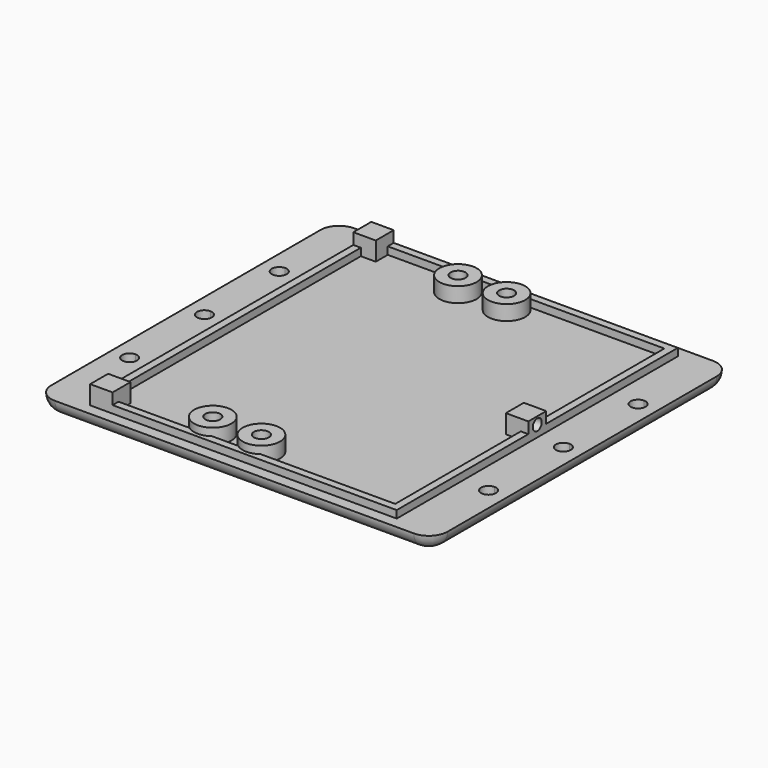
from build123d import *

# Parameters (mm, degrees)
F0_W          = 106
F0_H          = 100
F1_DEPTH      = 4
F2_W          = 82
F2_H          = 94
F2_W_2        = 78
F2_H_2        = 90
F5_DEPTH      = 2
F6_DEPTH      = 25
F4_R          = 5
F4_R_2        = 2
F7_DEPTH      = 4
F8_W          = 6
F8_H          = 6
F9_DEPTH      = 5
F10_R         = 1.5
F11_DEPTH     = 5
F12_W         = 6
F12_H         = 6
F13_DEPTH     = 5
F14_R         = 1.5
F15_DEPTH     = 5
F16_R         = 5
F17_T1_DEPTH  = 90
F17_T3_DEPTH  = 96
F17_T6_ANGLE  = 90
F17_T8_ANGLE  = 90
F17_T10_ANGLE = 90
F17_T12_ANGLE = 90


# Not quite as in the source:
# - a fillet or chamfer that OpenCascade refuses, or shapes differently, is made with other operations: its cross-section is extruded or revolved along the edge and cut away or added


with BuildPart() as f1:
    # F0 (on Top) → F1 (new body)
    with BuildSketch(Plane.XY):
        with Locations((-29.9393483698, 26.8405017372)):
            Rectangle(F0_W, F0_H)
    extrude(amount=F1_DEPTH)

    # F2 (on face) → F5 (join)
    with BuildSketch(Plane.XY.offset(4)):
        with Locations((-29.9393483698, 26.8405017372)):
            Rectangle(F2_W, F2_H)
        with Locations((-29.9393483698, 26.8405017372)):
            Rectangle(F2_W_2, F2_H_2, mode=Mode.SUBTRACT)
    extrude(amount=F5_DEPTH)

    # F3 (on face) → F6 (cut)
    with BuildSketch(Plane.XY.offset(4)):
        with BuildLine():
            ThreePointArc((-77.9393483698, 49.7999965698), (-76.5251348075, 50.3857830074), (-75.9393483698, 51.7999965698))
            ThreePointArc((-75.9393483698, 51.7999965698), (-76.5251348075, 53.2142101321), (-77.9393483698, 53.7999965698))
            Line((-77.9393483698, 53.7999965698), (-77.9393483698, 51.7999965698))
            Line((-77.9393483698, 51.7999965698), (-77.9393483698, 49.7999965698))
        make_face()
        with BuildLine():
            ThreePointArc((-75.9393483698, 1.7999965698), (-76.5251348075, 3.2142101321), (-77.9393483698, 3.7999965698))
            Line((-77.9393483698, 3.7999965698), (-77.9393483698, 1.7999965698))
            Line((-77.9393483698, 1.7999965698), (-77.9393483698, -0.2000034302))
            ThreePointArc((-77.9393483698, -0.2000034302), (-76.5251348075, 0.3857830074), (-75.9393483698, 1.7999965698))
        make_face()
        with BuildLine():
            Line((-77.9393483698, 1.7999965698), (-77.9393483698, 3.7999965698))
            ThreePointArc((-77.9393483698, 3.7999965698), (-79.9393483698, 1.7999965698), (-77.9393483698, -0.2000034302))
            Line((-77.9393483698, -0.2000034302), (-77.9393483698, 1.7999965698))
        make_face()
        with BuildLine():
            ThreePointArc((-75.9393483698, 26.7999965698), (-76.5251348075, 28.2142101321), (-77.9393483698, 28.7999965698))
            Line((-77.9393483698, 28.7999965698), (-77.9393483698, 26.7999965698))
            Line((-77.9393483698, 26.7999965698), (-77.9393483698, 24.7999965698))
            ThreePointArc((-77.9393483698, 24.7999965698), (-76.5251348075, 25.3857830074), (-75.9393483698, 26.7999965698))
        make_face()
        with BuildLine():
            Line((-77.9393483698, 26.7999965698), (-77.9393483698, 28.7999965698))
            ThreePointArc((-77.9393483698, 28.7999965698), (-79.9393483698, 26.7999965698), (-77.9393483698, 24.7999965698))
            Line((-77.9393483698, 24.7999965698), (-77.9393483698, 26.7999965698))
        make_face()
        with BuildLine():
            Line((-77.9393483698, 51.7999965698), (-77.9393483698, 53.7999965698))
            ThreePointArc((-77.9393483698, 53.7999965698), (-79.9393483698, 51.7999965698), (-77.9393483698, 49.7999965698))
            Line((-77.9393483698, 49.7999965698), (-77.9393483698, 51.7999965698))
        make_face()
        with BuildLine():
            ThreePointArc((18.0606516302, 49.7999965698), (19.4748651925, 50.3857830074), (20.0606516302, 51.7999965698))
            ThreePointArc((20.0606516302, 51.7999965698), (19.4748651925, 53.2142101321), (18.0606516302, 53.7999965698))
            Line((18.0606516302, 53.7999965698), (18.0606516302, 51.7999965698))
            Line((18.0606516302, 51.7999965698), (18.0606516302, 49.7999965698))
        make_face()
        with BuildLine():
            ThreePointArc((20.0606516302, 1.7999965698), (19.4748651925, 3.2142101321), (18.0606516302, 3.7999965698))
            ThreePointArc((18.0606516302, 3.7999965698), (16.6464380678, 0.3857830074), (20.0606516302, 1.7999965698))
        make_face()
        with BuildLine():
            ThreePointArc((20.0606516302, 26.7999965698), (19.4748651925, 28.2142101321), (18.0606516302, 28.7999965698))
            Line((18.0606516302, 28.7999965698), (18.0606516302, 26.7999965698))
            Line((18.0606516302, 26.7999965698), (18.0606516302, 24.7999965698))
            ThreePointArc((18.0606516302, 24.7999965698), (19.4748651925, 25.3857830074), (20.0606516302, 26.7999965698))
        make_face()
        with BuildLine():
            Line((18.0606516302, 26.7999965698), (18.0606516302, 28.7999965698))
            ThreePointArc((18.0606516302, 28.7999965698), (16.0606516302, 26.7999965698), (18.0606516302, 24.7999965698))
            Line((18.0606516302, 24.7999965698), (18.0606516302, 26.7999965698))
        make_face()
        with BuildLine():
            Line((18.0606516302, 51.7999965698), (18.0606516302, 53.7999965698))
            ThreePointArc((18.0606516302, 53.7999965698), (16.0606516302, 51.7999965698), (18.0606516302, 49.7999965698))
            Line((18.0606516302, 49.7999965698), (18.0606516302, 51.7999965698))
        make_face()
    extrude(amount=-F6_DEPTH, mode=Mode.SUBTRACT)

    # F4 (on face) → F7 (join)
    with BuildSketch(Plane.XY.offset(4)):
        with Locations((-42.9393483698, 67.8405017372)):
            Circle(F4_R)
        with Locations((-42.9393483698, 67.8405017372)):
            Circle(F4_R_2, mode=Mode.SUBTRACT)
        with Locations((-29.9393483698, 67.8405017372)):
            Circle(F4_R)
        with Locations((-29.9393483698, 67.8405017372)):
            Circle(F4_R_2, mode=Mode.SUBTRACT)
        with Locations((-42.9393483698, -14.1594982628)):
            Circle(F4_R)
        with Locations((-42.9393483698, -14.1594982628)):
            Circle(F4_R_2, mode=Mode.SUBTRACT)
        with Locations((-29.9393483698, -14.1594982628)):
            Circle(F4_R)
        with Locations((-29.9393483698, -14.1594982628)):
            Circle(F4_R_2, mode=Mode.SUBTRACT)
    extrude(amount=F7_DEPTH)

    # F8 (on face) → F9 (join)
    with BuildSketch(Plane.XY.offset(4)):
        with Locations((-67.9393483698, 70.8405017372)):
            Rectangle(F8_W, F8_H)
        with Locations((-67.9393483698, -17.1594982628)):
            Rectangle(F8_W, F8_H)
    extrude(amount=F9_DEPTH)

    # F10 (on face) → F11 (cut)
    with BuildSketch(Plane(origin=(-70.9393483698, 0, 0), x_dir=(0, -1, 0), z_dir=(-1, 0, 0))):
        with Locations((-70.8405017372, 7)):
            Circle(F10_R)
        with Locations((17.1594982628, 7)):
            Circle(F10_R)
    extrude(amount=-F11_DEPTH, mode=Mode.SUBTRACT)

    # F12 (on face) → F13 (join)
    with BuildSketch(Plane.XY.offset(4)):
        with Locations((8.0606516302, 26.8405017372)):
            Rectangle(F12_W, F12_H)
    extrude(amount=F13_DEPTH)

    # F14 (on face) → F15 (cut)
    with BuildSketch(Plane.YZ.offset(11.0606516302)):
        with Locations((26.8405017372, 7)):
            Circle(F14_R)
    extrude(amount=-F15_DEPTH, mode=Mode.SUBTRACT)

    # F16
    f16_edges = [f1.edges().sort_by_distance(p)[0] for p in [
        (-82.939348, 76.840502, 2),
        (23.060652, 76.840502, 2),
        (23.060652, -23.159498, 2),
        (-82.939348, -23.159498, 2),
    ]]
    fillet(f16_edges, radius=F16_R)

    # F17: fillet of radius 4 on 8 edges, made by hand

    # F17_s2 → F17_t1 (cut)
    with BuildSketch(Plane.XZ.offset(-71.8405017372)):
        with BuildLine():
            ThreePointArc((23.0606516302, 4), (21.8890787549, 1.1715728753), (19.0606516302, 0))
            Line((19.0606516302, 0), (23.0606516302, 0))
            Line((23.0606516302, 0), (23.0606516302, 4))
        make_face()
        with BuildLine():
            ThreePointArc((-78.9393483698, 0), (-81.7677754946, 1.1715728753), (-82.9393483698, 4))
            Line((-82.9393483698, 4), (-82.9393483698, 0))
            Line((-82.9393483698, 0), (-78.9393483698, 0))
        make_face()
    extrude(amount=F17_T1_DEPTH, mode=Mode.SUBTRACT)

    # F17_s4 → F17_t3 (cut)
    with BuildSketch(Plane.YZ.offset(-77.9393483698)):
        with BuildLine():
            ThreePointArc((-19.1594982628, 0), (-21.9879253875, 1.1715728753), (-23.1594982628, 4))
            Line((-23.1594982628, 4), (-23.1594982628, 0))
            Line((-23.1594982628, 0), (-19.1594982628, 0))
        make_face()
        with BuildLine():
            ThreePointArc((72.8405017372, 0), (75.668928862, 1.1715728753), (76.8405017372, 4))
            Line((76.8405017372, 4), (76.8405017372, 0))
            Line((76.8405017372, 0), (72.8405017372, 0))
        make_face()
    extrude(amount=F17_T3_DEPTH, mode=Mode.SUBTRACT)

    # F17_s5 → F17_t6 (revolve, cut)
    with BuildSketch(Plane.XZ.offset(18.1594982628)):
        with BuildLine():
            ThreePointArc((19.0606516302, 0), (21.8890787549, 1.1715728753), (23.0606516302, 4))
            Line((23.0606516302, 4), (23.0606516302, 0))
            Line((23.0606516302, 0), (19.0606516302, 0))
        make_face()
    revolve(axis=Axis((18.0606516302, -18.1594982628, 0), (0, 0, -1)), revolution_arc=F17_T6_ANGLE, mode=Mode.SUBTRACT)

    # F17_s7 → F17_t8 (revolve, cut)
    with BuildSketch(Plane.XZ.offset(-71.8405017372)):
        with BuildLine():
            ThreePointArc((19.0606516302, 0), (21.8890787549, 1.1715728753), (23.0606516302, 4))
            Line((23.0606516302, 4), (23.0606516302, 0))
            Line((23.0606516302, 0), (19.0606516302, 0))
        make_face()
    revolve(axis=Axis((18.0606516302, 71.8405017372, 0), (0, 0, 1)), revolution_arc=F17_T8_ANGLE, mode=Mode.SUBTRACT)

    # F17_s9 → F17_t10 (revolve, cut)
    with BuildSketch(Plane.YZ.offset(-77.9393483698)):
        with BuildLine():
            ThreePointArc((-19.1594982628, 0), (-21.9879253875, 1.1715728753), (-23.1594982628, 4))
            Line((-23.1594982628, 4), (-23.1594982628, 0))
            Line((-23.1594982628, 0), (-19.1594982628, 0))
        make_face()
    revolve(axis=Axis((-77.9393483698, -18.1594982628, 0), (0, 0, -1)), revolution_arc=F17_T10_ANGLE, mode=Mode.SUBTRACT)

    # F17_s11 → F17_t12 (revolve, cut)
    with BuildSketch(Plane.YZ.offset(-77.9393483698)):
        with BuildLine():
            ThreePointArc((72.8405017372, 0), (75.668928862, 1.1715728753), (76.8405017372, 4))
            Line((76.8405017372, 4), (76.8405017372, 0))
            Line((76.8405017372, 0), (72.8405017372, 0))
        make_face()
    revolve(axis=Axis((-77.9393483698, 71.8405017372, 0), (0, 0, 1)), revolution_arc=F17_T12_ANGLE, mode=Mode.SUBTRACT)


solid = f1.part
